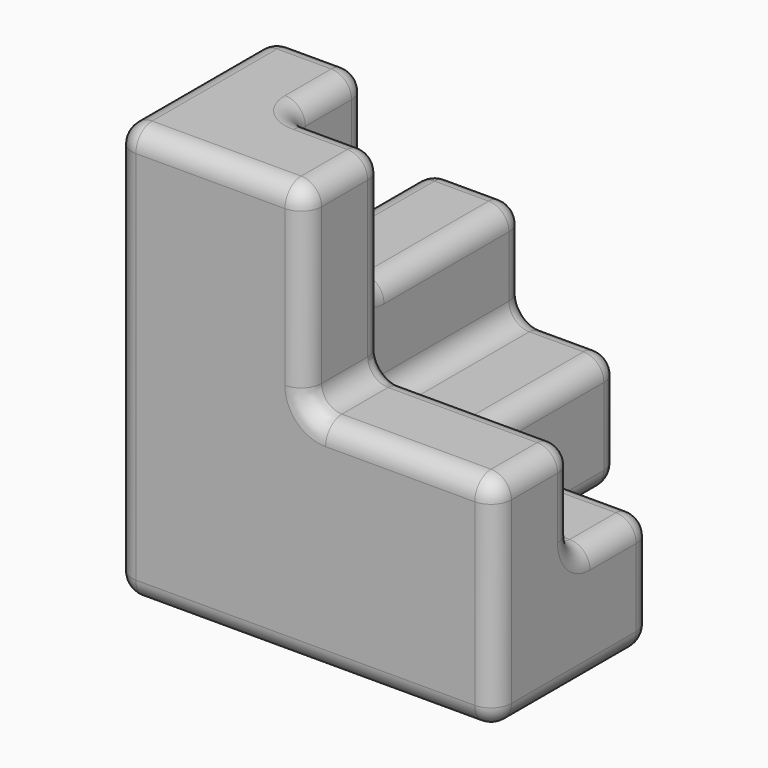
from build123d import *

# Parameters (mm, degrees)
F8_DEPTH  = 54.8865515739
F1_DEPTH  = 36.7471762002
F3_DEPTH  = 25.4
F10_DEPTH = 62.1797274798
F4_DEPTH  = 13.1793599576
F5_F1_R   = 5.08
F5_F2_R   = 5.08


with BuildPart() as f8:
    # F6 (on Top) → F8 (new body)
    with BuildSketch(Plane.XY):
        Polygon((-47.3731532693, 49.1066724062), (-47.3731532693, -49.1066724062), (47.3731532693, -49.1066724062), (47.3731532693, 0), (0, 0), (0, 49.1066724062), align=None)
    extrude(amount=F8_DEPTH)

    # F0 (on face) → F1 (join)
    with BuildSketch(Plane.XY.offset(54.8865515739)):
        Polygon((0, 49.1066724062), (-23.6865766346, 49.1066724062), (-23.6865766346, -24.5533362031), (47.3731532693, -24.5533362031), (47.3731532693, 0), (0, 0), align=None)
    extrude(amount=-F1_DEPTH)

    # F2 (on face) → F3 (cut)
    with BuildSketch(Plane.XY.offset(54.8865515739)):
        Polygon((-23.6865766346, -24.5533362031), (47.3731532693, -24.5533362031), (47.3731532693, 0), (0, 0), (0, 49.1066724062), (-23.6865766346, 49.1066724062), align=None)
    extrude(amount=-F3_DEPTH, mode=Mode.SUBTRACT)

    # F9 (on face) → F10 (join)
    with BuildSketch(Plane.XY.offset(54.8865515739)):
        Polygon((0, -49.1066724062), (-0.0103376806, -24.5533362031), (-23.6865766346, -24.5533362031), (-23.6865766346, -19.0210193396), (-23.6865766346, 0), (-47.3731532693, 0), (-47.3731532693, -11.8761584163), (-47.3731532693, -49.1066724062), align=None)
    extrude(amount=F10_DEPTH)

    # F4 (cut): a face of the model
    f4_faces = [f8.faces().sort_by_distance(p)[0] for p in [
        (-27.6363494072, -28.6452612162, 117.0662790537),
    ]]
    extrude(f4_faces, amount=-F4_DEPTH, mode=Mode.SUBTRACT)

    # F5: fillet of radius 5.08 on 32 edges, made by hand

    # F5_f1
    f5_f1_edges = [f8.edges().sort_by_distance(p)[0] for p in [
        (-23.6865766346, -24.5533362031, 66.686735335),
        (-35.529864952, 0, 54.8865515739),
        (-0.0051688403, -36.8300043046, 54.8865515739),
        (11.8432883173, -24.5533362031, 29.4865515739),
        (-23.6865766346, 12.2766681015, 29.4865515739),
    ]]
    fillet(f5_f1_edges, radius=F5_F1_R)

    # F5_f2
    f5_f2_edges = [f8.edges().sort_by_distance(p)[0] for p in [
        (-0.0051688403, -36.8300043046, 103.8869190961),
        (-9.3084571576, -24.5533362031, 103.8869190961),
        (-23.6865766346, -9.7366681015, 103.8869190961),
        (-35.529864952, 0, 103.8869190961),
        (-47.3731532693, -24.5533362031, 103.8869190961),
        (-23.6865766346, -49.1066724062, 103.8869190961),
        (-0.0103376806, -24.5533362031, 81.926735335),
        (0, -49.1066724062, 81.926735335),
        (-23.6865766346, 0, 81.926735335),
        (-47.3731532693, 0, 81.926735335),
        (47.3731532693, -36.8300043046, 54.8865515739),
        (-35.529864952, 49.1066724062, 54.8865515739),
        (23.6865766346, 0, 0),
        (47.3731532693, -24.5533362031, 0),
        (47.3731532693, 0, 14.7432757869),
        (23.6865766346, 0, 29.4865515739),
        (47.3731532693, -9.7366681015, 29.4865515739),
        (0, 24.5533362031, 29.4865515739),
        (-9.3032883173, 49.1066724062, 29.4865515739),
        (0, 49.1066724062, 14.7432757869),
        (0, 24.5533362031, 0),
        (47.3731532693, -49.1066724062, 27.4432757869),
        (0, -49.1066724062, 0),
        (-47.3731532693, -49.1066724062, 51.9434595481),
        (-23.6865766346, 49.1066724062, 0),
        (-47.3731532693, 49.1066724062, 27.4432757869),
        (-47.3731532693, 0, 0),
        (-22.1986790831, 49.1066724062, 30.9744491254),
        (47.3731532693, -23.0654386515, 30.9744491254),
        (-47.3731532693, 1.4878975516, 56.3744491254),
        (-23.6865766346, 1.4878975516, 56.3744491254),
        (1.4878976834, -49.1066724062, 56.3744491254),
        (1.4775600029, -24.5533362031, 56.3744491254),
        (-22.1986790831, -23.0654386515, 103.8869190961),
    ]]
    fillet(f5_f2_edges, radius=F5_F2_R)


solid = f8.part
